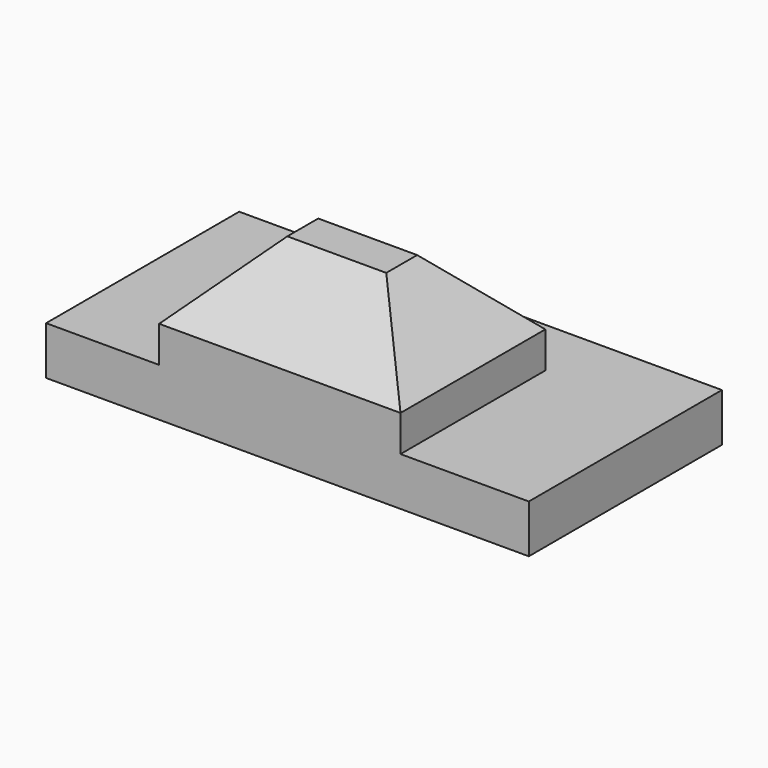
from build123d import *

# Parameters (mm, degrees)
F0_W      = 1016
F0_H      = 508
F1_DEPTH  = 101.6
F4_W      = 237.9516797066
F4_H      = 381
F4_W_2    = 270.0483202934
F5_DEPTH  = 76.2
F5_FACE_W = 508
F5_FACE_H = 381
F6_DEPTH  = 149.86
F6_TAPER  = 45
F8_DEPTH  = 76.2


# Not quite as in the source:
# - the program builds the solid bodies; features that only make, move or delete a surface that nothing else refers to are left out


with BuildPart() as f1:
    # F0 (on Top) → F1 (new body)
    with BuildSketch(Plane.XY):
        Rectangle(F0_W, F0_H)
    extrude(amount=F1_DEPTH)

    # F4 (on face) → F5 (join)
    with BuildSketch(Plane.XY.offset(101.6)):
        with Locations((118.9758398533, -63.5)):
            Rectangle(F4_W, F4_H)
        with Locations((-135.0241601467, -63.5)):
            Rectangle(F4_W_2, F4_H)
    extrude(amount=F5_DEPTH)

    # F5_face (on face) → F6 (join, symmetric)
    with BuildSketch(Plane(origin=(-16.0483202934, -63.5, 177.8), x_dir=(1, 0, 0), z_dir=(0, 0, 1))):
        Rectangle(F5_FACE_W, F5_FACE_H)
    extrude(amount=F6_DEPTH, both=True, taper=F6_TAPER)

    # F7 (on face) → F8 (cut)
    with BuildSketch(Plane(origin=(0, 152.4, 152.4), x_dir=(-1, 0, 0), z_dir=(0, 0.7071067812, 0.7071067812))):
        Polygon((-18.2156057455, 126.8785575445), (57.9806947666, 127.6294159035), (19.232282097, 193.2419186418), align=None)
    extrude(amount=-F8_DEPTH, mode=Mode.SUBTRACT)


solid = f1.part
